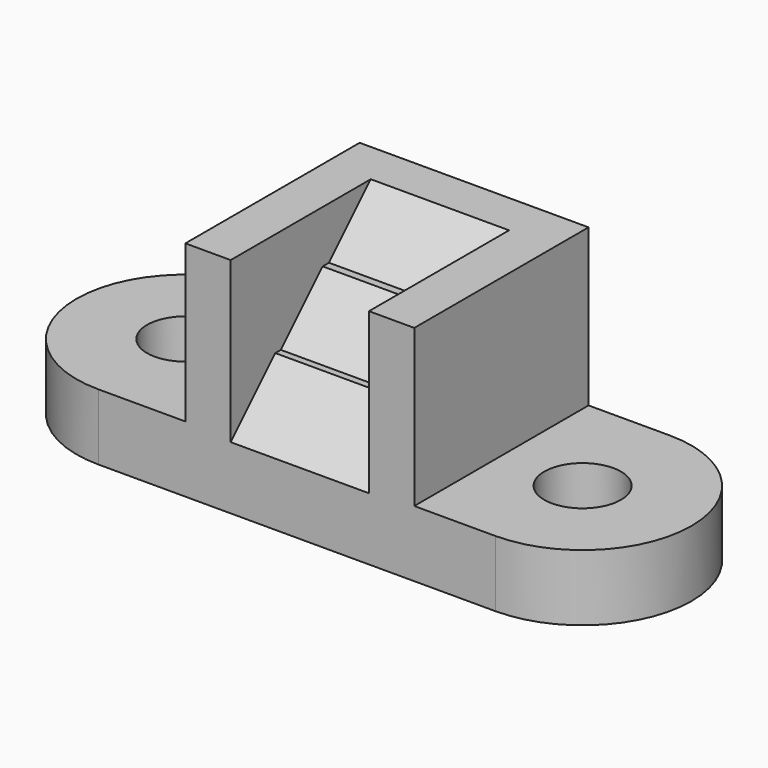
from build123d import *

# Parameters (mm, degrees)
F1_DEPTH     = 19
F2_R         = 11
F3_DEPTH     = 19
F5_DEPTH     = 45
F6_W         = 39.6946725957
F6_H         = 17
F7_DEPTH     = 15
F8_W         = 39.6946725957
F8_H         = 16.2631579523
F9_DEPTH     = 30
F10_T1_DEPTH = 39.6946725957
F10_T6_DEPTH = 39.6946725957
F11_W        = 39.6946725957
F11_H        = 16.2631579523
F12_DEPTH    = 45
F13_T4_DEPTH = 39.6946725957


# Not quite as in the source:
# - a fillet or chamfer that OpenCascade refuses, or shapes differently, is made with other operations: its cross-section is extruded or revolved along the edge and cut away or added


with BuildPart() as f1:
    # F0 (on Top) → F1 (new body)
    with BuildSketch(Plane.XY):
        with BuildLine():
            ThreePointArc((-107.8725005202, 54.8863680974), (-139.1356584725, 23.6232101452), (-107.8725005202, -7.6399478071))
            Line((-107.8725005202, -7.6399478071), (6.1274994798, -7.6399478071))
            ThreePointArc((6.1274994798, -7.6399478071), (37.3906574321, 23.6232101452), (6.1274994798, 54.8863680974))
            Line((6.1274994798, 54.8863680974), (-107.8725005202, 54.8863680974))
        make_face()
    extrude(amount=F1_DEPTH)

    # F2 (on face) → F3 (cut)
    with BuildSketch(Plane.XY.offset(19)):
        with Locations((-107.8725005202, 23.6232101452)):
            Circle(F2_R)
        with Locations((6.1274994798, 23.6232101452)):
            Circle(F2_R)
    extrude(amount=-F3_DEPTH, mode=Mode.SUBTRACT)

    # F4 (on face) → F5 (join)
    with BuildSketch(Plane.XY.offset(19)):
        Polygon((-17.1778279245, 54.8863680974), (-82.8725005202, 54.8863680974), (-82.8725005202, -7.6399478071), (-69.8725005202, -7.6399478071), (-69.8725005202, 41.8863680974), (-30.1778279245, 41.8863680974), (-30.1778279245, -7.6399478071), (-17.1778279245, -7.6399478071), align=None)
    extrude(amount=F5_DEPTH)

    # F6 (on face) → F7 (join)
    with BuildSketch(Plane.XY.offset(19)):
        with Locations((-50.0251642223, 0.8600521929)):
            Rectangle(F6_W, F6_H)
    extrude(amount=F7_DEPTH)

    # F8 (on face) → F9 (join)
    with BuildSketch(Plane.XY.offset(19)):
        with Locations((-50.0251642223, 17.491631169)):
            Rectangle(F8_W, F8_H)
    extrude(amount=F9_DEPTH)

    # F10: chamfer of 16 on 2 edges, made by hand

    # F10_s2 → F10_t1 (cut)
    with BuildSketch(Plane.YZ.offset(-69.8725005202)):
        Polygon((-7.6399478071, 18), (8.3600521929, 34), (-7.6399478071, 34), align=None)
    extrude(amount=F10_T1_DEPTH, mode=Mode.SUBTRACT)


with BuildPart() as f10_tool4:
    # F10_s5 → F10_t6 (new body)
    with BuildSketch(Plane.YZ.offset(-69.8725005202)):
        Polygon((9.3600521929, 33), (25.3600521929, 49), (9.3600521929, 49), align=None)
    extrude(amount=F10_T6_DEPTH)

    split(bisect_by=Plane.XY.offset(34), keep=Keep.TOP)


with BuildPart() as f1_1:
    add(f1.part)

    # F10_t3: cut F10_tool4
    add(f10_tool4.part, mode=Mode.SUBTRACT)

    # F11 (on face) → F12 (join)
    with BuildSketch(Plane.XY.offset(19)):
        with Locations((-50.0251642223, 33.7547891213)):
            Rectangle(F11_W, F11_H)
    extrude(amount=F12_DEPTH)

    # F13: chamfer of 17 on 1 edges, made by hand


with BuildPart() as f13_tool2:
    # F13_s3 → F13_t4 (new body)
    with BuildSketch(Plane.YZ.offset(-69.8725005202)):
        Polygon((42.6232101452, 64), (25.6232101452, 47), (25.6232101452, 64), align=None)
    extrude(amount=F13_T4_DEPTH)

    split(bisect_by=Plane.XY.offset(49), keep=Keep.TOP)


with BuildPart() as f1_2:
    add(f1_1.part)

    # F13_t1: cut F13_tool2
    add(f13_tool2.part, mode=Mode.SUBTRACT)


solid = f1_2.part
